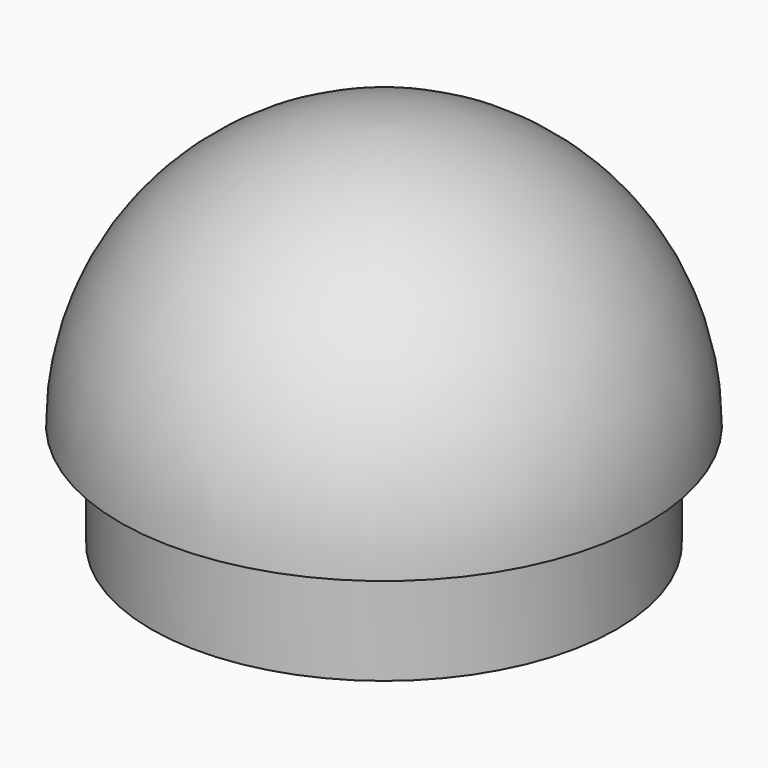
from build123d import *

# Parameters (mm, degrees)
F0_R     = 21.2725
F1_DEPTH = 9.525
F2_R     = 24.13
F3_DEPTH = 24.13
F4_R     = 24.12999


# Not quite as in the source:
# - a fillet or chamfer is up to 0.001 mm smaller than in the source, because OpenCascade refuses the exact size


with BuildPart() as f1:
    # F0 (on Top) → F1 (new body)
    with BuildSketch(Plane.XY):
        Circle(F0_R)
    extrude(amount=F1_DEPTH)

    # F2 (on face) → F3 (join)
    with BuildSketch(Plane.XY.offset(9.525)):
        Circle(F2_R)
    extrude(amount=F3_DEPTH)

    # F4 (radius 24.13 in the source; OpenCascade refuses exactly that, so slightly less here)
    f4_edges = [f1.edges().sort_by_distance(p)[0] for p in [
        (-24.13, 0, 33.655),
    ]]
    fillet(f4_edges, radius=F4_R)


solid = f1.part
